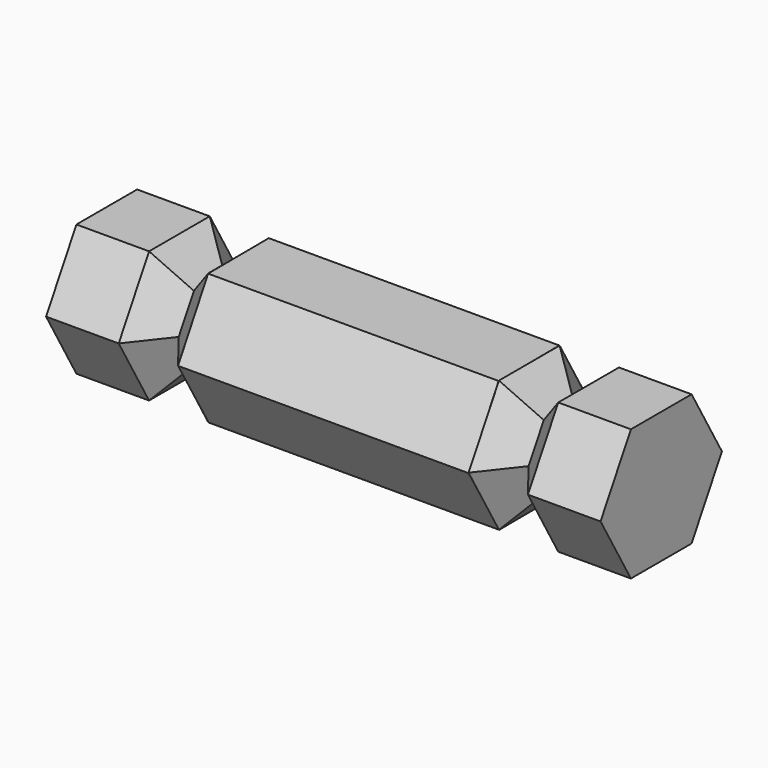
from build123d import *

# Parameters (mm, degrees)
F1_DEPTH = 30
F4_DEPTH = 60


with BuildPart() as f1:
    # F0 (on Right) → F1 (new body)
    with BuildSketch(Plane.YZ):
        Polygon((15.664, -27.1308438498), (31.328, 0), (15.664, 27.1308438498), (-15.664, 27.1308438498), (-31.328, 0), (-15.664, -27.1308438498), align=None)
    extrude(amount=F1_DEPTH)



with BuildPart() as f4:
    # F3 (on offset) → F4 (new body)
    with BuildSketch(Plane.YZ.offset(-24.5)):
        Polygon((15.8121267025, -27.0447819948), (31.3275315985, 0.1713124148), (15.515404896, 27.2160944096), (-15.8121267025, 27.0447819948), (-31.3275315985, -0.1713124148), (-15.515404896, -27.2160944096), align=None)
    extrude(amount=-F4_DEPTH)


with BuildPart() as f1_1:
    add(f1.part)

    add(f4.part)  # F8 merges F4
    # F6 (on Right) → F8 section 0
    with BuildSketch(Plane.YZ, mode=Mode.PRIVATE) as f8_s0:
        Polygon((15.664, -27.1308438498), (31.328, 0), (15.664, 27.1308438498), (-15.664, 27.1308438498), (-31.328, 0), (-15.664, -27.1308438498), align=None)
    loft([f8_s0.sketch, Vertex(-24.5, 0, 0)])

    # F7 (on offset) → F9 section 0
    with BuildSketch(Plane.YZ.offset(-24.5), mode=Mode.PRIVATE) as f9_s0:
        Polygon((15.664, -27.1308438498), (31.328, 0), (15.664, 27.1308438498), (-15.664, 27.1308438498), (-31.328, 0), (-15.664, -27.1308438498), align=None)
    loft([f9_s0.sketch, Vertex(0, 0, 0)])

    # F10: F1 across plane


with BuildPart() as f1_2:
    add(f1_1.part)
    add(f1_1.part.mirror(Plane(origin=(-84.5, 0, 0), x_dir=(0, 1, 0), z_dir=(-1, 0, 0))))


solid = f1_2.part
